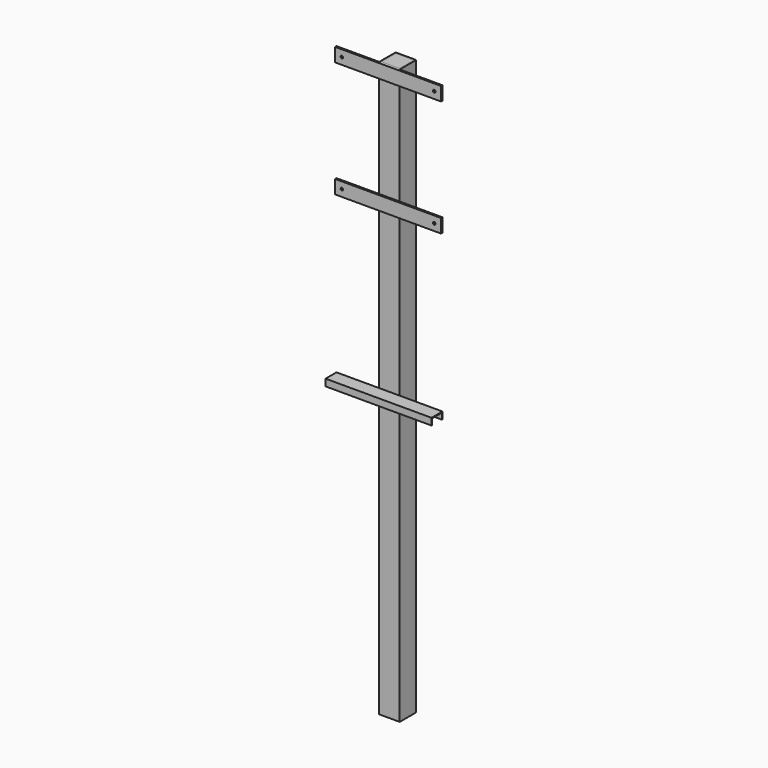
from build123d import *

# Parameters (mm, degrees)
F0_W          = 76.2
F0_H          = 76.2
F0_W_2        = 66.675
F0_H_2        = 66.675
F1_DEPTH      = 2133.6
F2_W          = 66.675
F2_H          = 66.675
F4_DEPTH      = 4.7625
F5_W          = 158.75
F5_H          = 50.8105754852
F5_R          = 4.7625
F5_W_2        = 76.2
F5_H_2        = 50.8
F6_DEPTH      = 6.35
F8_DEPTH      = 158.75
F8_DEPTH_BACK = 234.95


# Not quite as in the source:
# - a feature names something its author has since deleted; it is built from what else it names


with BuildPart() as f1:
    # F0 (on Top) → F1 (new body)
    with BuildSketch(Plane.XY):
        with Locations((-0.0228539575, -0.3835560492)):
            Rectangle(F0_W, F0_H)
        with Locations((-0.0228539575, -0.3835560492)):
            Rectangle(F0_W_2, F0_H_2, mode=Mode.SUBTRACT)
    extrude(amount=F1_DEPTH)

    # F5 (on face) → F6 (join)
    with BuildSketch(Plane.XZ.offset(38.4835560492)):
        with Locations((-117.4978539575, 1676.3947122574)):
            Rectangle(F5_W, F5_H)
        with Locations((-171.4728539575, 1676.4)):
            Circle(F5_R, mode=Mode.SUBTRACT)
        with Locations((117.4521460425, 1676.3947122574)):
            Rectangle(F5_W, F5_H)
        with Locations((171.4271460425, 1676.4)):
            Circle(F5_R, mode=Mode.SUBTRACT)
        with Locations((-0.0228539575, 1676.3947122574)):
            Rectangle(F5_W_2, F5_H)
        with Locations((-117.4978539575, 2108.2)):
            Rectangle(F5_W, F5_H_2)
        with Locations((-171.4728539575, 2108.2)):
            Circle(F5_R, mode=Mode.SUBTRACT)
        with Locations((-0.0228539575, 2108.2)):
            Rectangle(F5_W_2, F5_H_2)
        with Locations((117.4521460425, 2108.2)):
            Rectangle(F5_W, F5_H_2)
        with Locations((171.4271460425, 2108.2)):
            Circle(F5_R, mode=Mode.SUBTRACT)
    extrude(amount=F6_DEPTH)


with BuildPart() as f4:
    # F2 (on face) → F4 (new body)
    with BuildSketch(Plane.XY.offset(2133.6)):
        with Locations((-0.0228539575, -0.3835560492)):
            Rectangle(F2_W, F2_H)
    extrude(amount=-F4_DEPTH)


with BuildPart() as f8:
    # F7 (on face) → F8 (new body, two sides)
    with BuildSketch(Plane.YZ.offset(38.0771460425)) as f8_sk:
        Polygon((-38.4835560492, 1041.4), (-38.4835560492, 1066.8), (-89.2835560492, 1066.8), (-89.2835560492, 1041.4), (-86.1085560492, 1041.4), (-86.1085560492, 1063.625), (-41.6585560492, 1063.625), (-41.6585560492, 1041.4), align=None)
    extrude(amount=F8_DEPTH)
    extrude(f8_sk.sketch, amount=-F8_DEPTH_BACK)


solid = Compound([f1.part, f4.part, f8.part])
